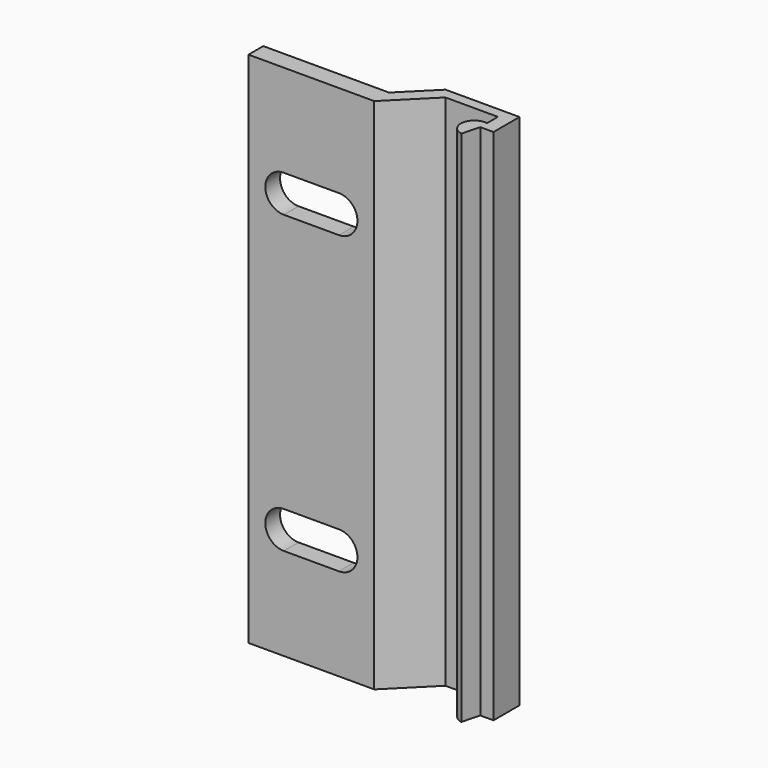
from build123d import *

# Parameters (mm, degrees)
F1_DEPTH = 88.9
F3_DEPTH = 25.4
F4_ANGLE = -90


with BuildPart() as f1:
    # F0 (on Front) → F1 (new body)
    with BuildSketch(Plane.XZ):
        Polygon((21.59, 0), (0, 0), (0, -3.175), (21.59, -3.175), (28.3751536726, 3.6101536726), (37.3921536726, 3.6101536726), (37.3921536726, 1.256122898), (36.5982342043, -3.2464181487), (37.4145606636, -0.1998463274), (39.6781536726, -0.1998463274), (39.6781536726, 5.3881536726), (26.9781536726, 5.3881536726), align=None)
        with BuildLine():
            Line((36.5982342043, -3.2464181487), (37.3921536726, 1.256122898))
            ThreePointArc((37.3921536726, 1.256122898), (34.7439234151, -0.5981878912), (36.5982342043, -3.2464181487))
        make_face()
    extrude(amount=F1_DEPTH)

    # F2 (on face) → F3 (cut)
    with BuildSketch(Plane.XY):
        with BuildLine():
            Line((10.795, -22.225), (10.795, -15.875))
            Line((10.795, -15.875), (6.06425, -15.875))
            ThreePointArc((6.06425, -15.875), (2.88925, -19.05), (6.06425, -22.225))
            Line((6.06425, -22.225), (10.795, -22.225))
        make_face()
        with BuildLine():
            Line((15.52575, -15.875), (10.795, -15.875))
            Line((10.795, -15.875), (10.795, -22.225))
            Line((10.795, -22.225), (15.52575, -22.225))
            ThreePointArc((15.52575, -22.225), (18.70075, -19.05), (15.52575, -15.875))
        make_face()
        with BuildLine():
            Line((10.795, -73.025), (10.795, -66.675))
            Line((10.795, -66.675), (6.06425, -66.675))
            ThreePointArc((6.06425, -66.675), (2.88925, -69.85), (6.06425, -73.025))
            Line((6.06425, -73.025), (10.795, -73.025))
        make_face()
        with BuildLine():
            Line((15.52575, -66.675), (10.795, -66.675))
            Line((10.795, -66.675), (10.795, -73.025))
            Line((10.795, -73.025), (15.52575, -73.025))
            ThreePointArc((15.52575, -73.025), (18.70075, -69.85), (15.52575, -66.675))
        make_face()
    extrude(amount=-F3_DEPTH, mode=Mode.SUBTRACT)


with BuildPart() as f1_1:
    # F4: moved
    add(f1.part.rotate(Axis((10.795, 0, 0), (1, 0, 0)), F4_ANGLE))


solid = f1_1.part
